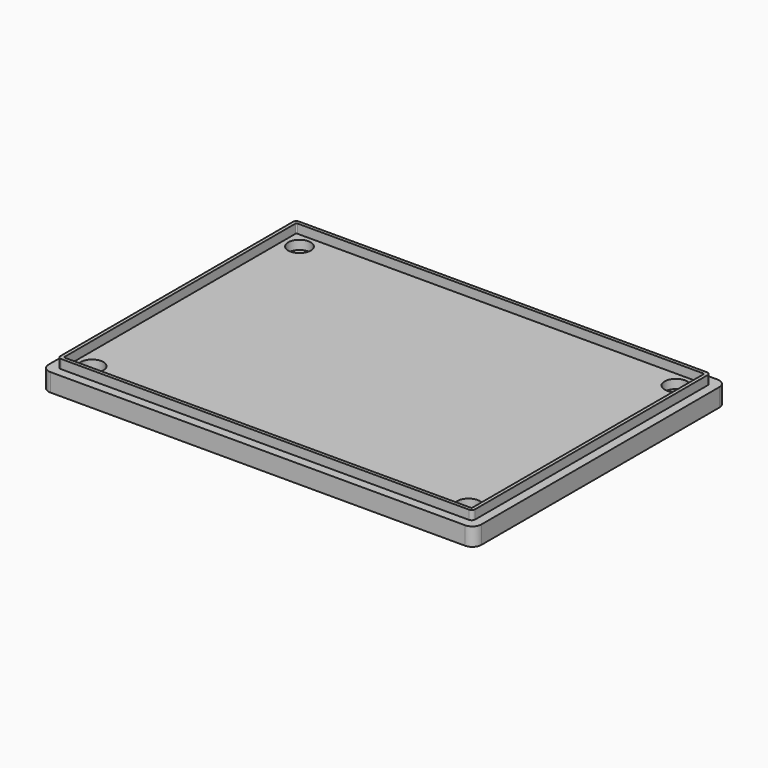
from build123d import *

# Parameters (mm, degrees)
F1_DEPTH  = 26
F2_DEPTH  = 4
F3_W      = 90
F3_H      = 64
F4_DEPTH  = 2
F6_DEPTH  = 2
F7_R      = 2.5
F8_DEPTH  = 2
F9_R      = 2.5
F10_DEPTH = 2
F11_W     = 5
F11_H     = 50
F11_W_2   = 76
F11_H_2   = 5
F12_DEPTH = 22
F13_R     = 1
F14_DEPTH = 5
F15_R     = 11
F15_R_2   = 5
F16_DEPTH = 2
F17_DEPTH = 5
F19_W     = 20.16
F19_H     = 11.52
F19_R     = 3
F19_R_2   = 2
F20_DEPTH = 5
F19_W_2   = 66
F19_H_2   = 18
F19_R_3   = 1.8
F21_DEPTH = 3
F22_DEPTH = 3
F19_R_4   = 0.8
F23_DEPTH = 1.9
F24_DEPTH = 1.9
F25_DEPTH = 1.9


# Not quite as in the source:
# - a feature names something its author has since deleted; it is built from what else it names


with BuildPart() as f1:
    # F0 (on Top) → F1 (new body)
    with BuildSketch(Plane.XY):
        with BuildLine():
            Line((46, 35), (-46, 35))
            ThreePointArc((-46, 35), (-47.4142135624, 34.4142135624), (-48, 33))
            Line((-48, 33), (-48, -33))
            ThreePointArc((-48, -33), (-47.4142135624, -34.4142135624), (-46, -35))
            Line((-46, -35), (46, -35))
            ThreePointArc((46, -35), (47.4142135624, -34.4142135624), (48, -33))
            Line((48, -33), (48, 33))
            ThreePointArc((48, 33), (47.4142135624, 34.4142135624), (46, 35))
        make_face()
    extrude(amount=F1_DEPTH)


with BuildPart() as f2:
    # F2 (new): a face of the model
    f2_faces = [f1.part.faces().sort_by_distance(p)[0] for p in [
        (0, 0, 26),
    ]]
    extrude(f2_faces, amount=F2_DEPTH)

    # F5 (on face) → F6 (join)
    with BuildSketch(Plane.XY.offset(30)):
        with BuildLine():
            Line((45.25, 33), (-45.25, 33))
            ThreePointArc((-45.25, 33), (-45.7803300859, 32.7803300859), (-46, 32.25))
            Line((-46, 32.25), (-46, -32.25))
            ThreePointArc((-46, -32.25), (-45.7803300859, -32.7803300859), (-45.25, -33))
            Line((-45.25, -33), (45.25, -33))
            ThreePointArc((45.25, -33), (45.7803300859, -32.7803300859), (46, -32.25))
            Line((46, -32.25), (46, 32.25))
            ThreePointArc((46, 32.25), (45.7803300859, 32.7803300859), (45.25, 33))
        make_face()
        with BuildLine():
            ThreePointArc((-45.25, 32), (-45.1767766953, 32.1767766953), (-45, 32.25))
            Line((-45, 32.25), (45, 32.25))
            ThreePointArc((45, 32.25), (45.1767766953, 32.1767766953), (45.25, 32))
            Line((45.25, 32), (45.25, -32))
            ThreePointArc((45.25, -32), (45.1767766953, -32.1767766953), (45, -32.25))
            Line((45, -32.25), (-45, -32.25))
            ThreePointArc((-45, -32.25), (-45.1767766953, -32.1767766953), (-45.25, -32))
            Line((-45.25, -32), (-45.25, 32))
        make_face(mode=Mode.SUBTRACT)
    extrude(amount=F6_DEPTH)

    # F9 (on face) → F10 (cut)
    with BuildSketch(Plane.XY.offset(30)):
        with Locations((-41.75, -28.75)):
            Circle(F9_R)
        with Locations((-41.75, 28.75)):
            Circle(F9_R)
        with Locations((41.75, 28.75)):
            Circle(F9_R)
        with Locations((41.75, -28.75)):
            Circle(F9_R)
    extrude(amount=-F10_DEPTH, mode=Mode.SUBTRACT)


with BuildPart() as f1_1:
    add(f1.part)

    # F3 (on face) → F4 (cut)
    with BuildSketch(Plane.XY.offset(26)):
        with BuildLine():
            Line((45, 33), (-45, 33))
            ThreePointArc((-45, 33), (-45.7071067812, 32.7071067812), (-46, 32))
            Line((-46, 32), (-46, -32))
            ThreePointArc((-46, -32), (-45.7071067812, -32.7071067812), (-45, -33))
            Line((-45, -33), (45, -33))
            ThreePointArc((45, -33), (45.7071067812, -32.7071067812), (46, -32))
            Line((46, -32), (46, 32))
            ThreePointArc((46, 32), (45.7071067812, 32.7071067812), (45, 33))
        make_face()
        Rectangle(F3_W, F3_H, mode=Mode.SUBTRACT)
    extrude(amount=-F4_DEPTH, mode=Mode.SUBTRACT)

    # F7 (on face) → F8 (cut)
    with BuildSketch(Plane.XY.offset(26)):
        with Locations((-41.5, -28.5)):
            Circle(F7_R)
        with Locations((-41.4999984205, 28.5)):
            Circle(F7_R)
        with Locations((41.5, 28.5)):
            Circle(F7_R)
        with Locations((41.5, -28.5)):
            Circle(F7_R)
    extrude(amount=-F8_DEPTH, mode=Mode.SUBTRACT)

    # F11 (on face) → F12 (cut)
    with BuildSketch(Plane.XY.offset(26)):
        with Locations((-40.5, 0)):
            Rectangle(F11_W, F11_H)
        with Locations((0, -27.5)):
            Rectangle(F11_W_2, F11_H_2)
        Rectangle(F11_W_2, F11_H)
        with Locations((0, 27.5)):
            Rectangle(F11_W_2, F11_H_2)
        with Locations((40.5, 0)):
            Rectangle(F11_W, F11_H)
    extrude(amount=-F12_DEPTH, mode=Mode.SUBTRACT)

    # F13 (on face) → F14 (cut, through all)
    with BuildSketch(Plane.YZ.offset(48)):
        with Locations((7.9999985173, 14.5000000224)):
            Circle(F13_R)
        with Locations((7.9999985173, 11.5000000224)):
            Circle(F13_R)
        with Locations((10.9999985173, 11.5000000224)):
            Circle(F13_R)
        with Locations((10.9999985173, 14.5000000224)):
            Circle(F13_R)
        with Locations((13.9999985173, 14.5000000224)):
            Circle(F13_R)
        with Locations((13.9999985173, 11.5000000224)):
            Circle(F13_R)
    extrude(amount=-F14_DEPTH, mode=Mode.SUBTRACT)

    # F15 (on face) → F16 (cut)
    with BuildSketch(Plane(origin=(-48, 0, 0), x_dir=(0, -1, 0), z_dir=(-1, 0, 0))):
        with Locations((6.9999988191, 12.5000002682)):
            Circle(F15_R)
        with Locations((6.9999988191, 12.5000002682)):
            Circle(F15_R_2, mode=Mode.SUBTRACT)
    extrude(amount=-F16_DEPTH, mode=Mode.SUBTRACT)

    # F15 (on face) → F17 (cut, through all)
    with BuildSketch(Plane(origin=(-48, 0, 0), x_dir=(0, -1, 0), z_dir=(-1, 0, 0))):
        with Locations((6.9999988191, 12.5000002682)):
            Circle(F15_R_2)
    extrude(amount=-F17_DEPTH, mode=Mode.SUBTRACT)

    # F19 (on face) → F20 (cut, through all)
    with BuildSketch(Plane(origin=(0, -30, 0), x_dir=(-1, 0, 0), z_dir=(0, 1, 0))):
        with Locations((4.7299169147, 14.0678631142)):
            Rectangle(F19_W, F19_H)
        with Locations((28.8399169147, 14.0678631142)):
            Circle(F19_R)
        with Locations((-11.1500830853, 14.0678631142)):
            Circle(F19_R_2)
        with Locations((-17.7100830853, 14.0678631142)):
            Circle(F19_R_2)
        with Locations((-24.2600830853, 14.0678631142)):
            Circle(F19_R_2)
        with BuildLine():
            ThreePointArc((-30.8900830853, 11.0678631142), (-30.5971898665, 10.360756333), (-29.8900830853, 10.0678631142))
            Line((-29.8900830853, 10.0678631142), (-28.9900830853, 10.0678631142))
            ThreePointArc((-28.9900830853, 10.0678631142), (-28.2829763041, 10.360756333), (-27.9900830853, 11.0678631142))
            Line((-27.9900830853, 11.0678631142), (-27.9900830853, 17.0678631142))
            ThreePointArc((-27.9900830853, 17.0678631142), (-28.2829763041, 17.7749698954), (-28.9900830853, 18.0678631142))
            Line((-28.9900830853, 18.0678631142), (-29.8900830853, 18.0678631142))
            ThreePointArc((-29.8900830853, 18.0678631142), (-30.5971898665, 17.7749698954), (-30.8900830853, 17.0678631142))
            Line((-30.8900830853, 17.0678631142), (-30.8900830853, 11.0678631142))
        make_face()
    extrude(amount=-F20_DEPTH, mode=Mode.SUBTRACT)

    # F19 (on face) → F21 (cut)
    with BuildSketch(Plane(origin=(0, -30, 0), x_dir=(-1, 0, 0), z_dir=(0, 1, 0))):
        with Locations((-0.1600830853, 14.0678631142)):
            Rectangle(F19_W_2, F19_H_2)
        with Locations((-24.0000830853, 7.5678631142)):
            Circle(F19_R_3, mode=Mode.SUBTRACT)
        with BuildLine():
            Line((-28.9900830853, 10.0678631142), (-29.8900830853, 10.0678631142))
            ThreePointArc((-29.8900830853, 10.0678631142), (-30.5971898665, 10.360756333), (-30.8900830853, 11.0678631142))
            Line((-30.8900830853, 11.0678631142), (-30.8900830853, 17.0678631142))
            ThreePointArc((-30.8900830853, 17.0678631142), (-30.5971898665, 17.7749698954), (-29.8900830853, 18.0678631142))
            Line((-29.8900830853, 18.0678631142), (-28.9900830853, 18.0678631142))
            ThreePointArc((-28.9900830853, 18.0678631142), (-28.2829763041, 17.7749698954), (-27.9900830853, 17.0678631142))
            Line((-27.9900830853, 17.0678631142), (-27.9900830853, 11.0678631142))
            ThreePointArc((-27.9900830853, 11.0678631142), (-28.2829763041, 10.360756333), (-28.9900830853, 10.0678631142))
        make_face(mode=Mode.SUBTRACT)
        with Locations((-24.2600830853, 14.0678631142)):
            Circle(F19_R_2, mode=Mode.SUBTRACT)
        with Locations((-17.7100830853, 14.0678631142)):
            Circle(F19_R_2, mode=Mode.SUBTRACT)
        with Locations((-11.1500830853, 14.0678631142)):
            Circle(F19_R_2, mode=Mode.SUBTRACT)
        with Locations((30.1799169147, 7.5678631142)):
            Circle(F19_R_3, mode=Mode.SUBTRACT)
        with Locations((4.7299169147, 14.0678631142)):
            Rectangle(F19_W, F19_H, mode=Mode.SUBTRACT)
        with Locations((28.8399169147, 14.0678631142)):
            Circle(F19_R, mode=Mode.SUBTRACT)
        with Locations((30.1799169147, 20.5678631142)):
            Circle(F19_R_3, mode=Mode.SUBTRACT)
    extrude(amount=F21_DEPTH, mode=Mode.SUBTRACT)

    # F19 (on face) → F22 (cut)
    with BuildSketch(Plane(origin=(0, -30, 0), x_dir=(-1, 0, 0), z_dir=(0, 1, 0))):
        with Locations((-0.1600830853, 14.0678631142)):
            Rectangle(F19_W_2, F19_H_2)
        with Locations((-24.0000830853, 7.5678631142)):
            Circle(F19_R_3, mode=Mode.SUBTRACT)
        with BuildLine():
            Line((-28.9900830853, 10.0678631142), (-29.8900830853, 10.0678631142))
            ThreePointArc((-29.8900830853, 10.0678631142), (-30.5971898665, 10.360756333), (-30.8900830853, 11.0678631142))
            Line((-30.8900830853, 11.0678631142), (-30.8900830853, 17.0678631142))
            ThreePointArc((-30.8900830853, 17.0678631142), (-30.5971898665, 17.7749698954), (-29.8900830853, 18.0678631142))
            Line((-29.8900830853, 18.0678631142), (-28.9900830853, 18.0678631142))
            ThreePointArc((-28.9900830853, 18.0678631142), (-28.2829763041, 17.7749698954), (-27.9900830853, 17.0678631142))
            Line((-27.9900830853, 17.0678631142), (-27.9900830853, 11.0678631142))
            ThreePointArc((-27.9900830853, 11.0678631142), (-28.2829763041, 10.360756333), (-28.9900830853, 10.0678631142))
        make_face(mode=Mode.SUBTRACT)
        with Locations((-24.2600830853, 14.0678631142)):
            Circle(F19_R_2, mode=Mode.SUBTRACT)
        with Locations((-17.7100830853, 14.0678631142)):
            Circle(F19_R_2, mode=Mode.SUBTRACT)
        with Locations((-11.1500830853, 14.0678631142)):
            Circle(F19_R_2, mode=Mode.SUBTRACT)
        with Locations((30.1799169147, 7.5678631142)):
            Circle(F19_R_3, mode=Mode.SUBTRACT)
        with Locations((4.7299169147, 14.0678631142)):
            Rectangle(F19_W, F19_H, mode=Mode.SUBTRACT)
        with Locations((28.8399169147, 14.0678631142)):
            Circle(F19_R, mode=Mode.SUBTRACT)
        with Locations((30.1799169147, 20.5678631142)):
            Circle(F19_R_3, mode=Mode.SUBTRACT)
    extrude(amount=-F22_DEPTH, mode=Mode.SUBTRACT)

    # F19 (on face) → F23 (join)
    with BuildSketch(Plane(origin=(0, -30, 0), x_dir=(-1, 0, 0), z_dir=(0, 1, 0))):
        with Locations((30.1799169147, 20.5678631142)):
            Circle(F19_R_3)
        with Locations((30.1799169147, 20.5678631142)):
            Circle(F19_R_4, mode=Mode.SUBTRACT)
    extrude(amount=F23_DEPTH)

    # F19 (on face) → F24 (join)
    with BuildSketch(Plane(origin=(0, -30, 0), x_dir=(-1, 0, 0), z_dir=(0, 1, 0))):
        with Locations((30.1799169147, 7.5678631142)):
            Circle(F19_R_3)
        with Locations((30.1799169147, 7.5678631142)):
            Circle(F19_R_4, mode=Mode.SUBTRACT)
    extrude(amount=F24_DEPTH)

    # F19 (on face) → F25 (join)
    with BuildSketch(Plane(origin=(0, -30, 0), x_dir=(-1, 0, 0), z_dir=(0, 1, 0))):
        with Locations((-24.0000830853, 7.5678631142)):
            Circle(F19_R_3)
        with Locations((-24.0000830853, 7.5678631142)):
            Circle(F19_R_4, mode=Mode.SUBTRACT)
    extrude(amount=F25_DEPTH)


with BuildPart() as f27_1:
    # F27: copy of F2
    add(f2.part)


with BuildPart() as f29_1:
    # F29: copy of F2
    add(f2.part)


solid = f2.part
